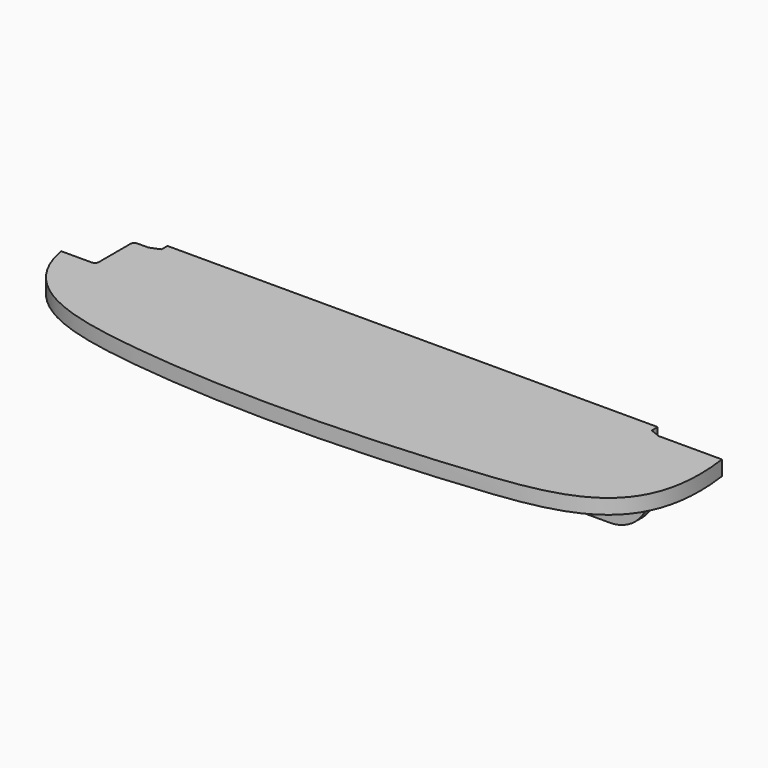
from build123d import *

# Parameters (mm, degrees)
F1_DEPTH = 19.05
F3_DEPTH = 25.4
F4_W     = 625.475
F4_H     = 11.1125
F5_DEPTH = 101.6
F6_R     = 50.8
F7_R     = 5.08


with BuildPart() as f1:
    # F0 (on Top) → F1 (new body)
    with BuildSketch(Plane.XY):
        with BuildLine():
            Line((398.4625, 0), (-398.4625, 0))
            Line((-398.4625, 0), (-398.4625, -75.40625))
            add(Edge.make_bspline(
                [(-398.4625, -75.40625), (-382.7767657486, -158.8698293815), (-186.1213914705, -212.4356276363), (207.7106026788, -201.6622700018), (427.1077817692, -162.9815576871), (398.4625, 0)],
                knots=[0.0603535709, 0.0603535709, 0.0603535709, 0.0603535709, 0.3014904815, 0.6985095185, 1, 1, 1, 1], degree=3))
        make_face()
    extrude(amount=F1_DEPTH)

    # F2 (on face) → F3 (cut)
    with BuildSketch(Plane.XY.offset(19.05)):
        Polygon((-322.1280574799, 0), (-398.4625, 0), (-398.4625, -75.40625), (-354.0125, -75.40625), (-354.0125, -14.684375), (-334.9625, -14.684375), (-322.2625, -9.525), align=None)
        Polygon((398.4625, 0), (382.8563850403, 0), (306.5219425201, 0), (306.6563850403, -9.525), (319.3563850403, -14.684375), (338.4063850403, -14.684375), (402.6769697666, -14.684375), align=None)
    extrude(amount=-F3_DEPTH, mode=Mode.SUBTRACT)

    # F7
    f7_edges = [f1.edges().sort_by_distance(p)[0] for p in [
        (-354.0125, -75.40625, 9.525),
        (-354.0125, -14.684375, 9.525),
    ]]
    fillet(f7_edges, radius=F7_R)


with BuildPart() as f5:
    # F4 (on Top) → F5 (new body)
    with BuildSketch(Plane.XY):
        with Locations((-7.8030574799, -5.55625)):
            Rectangle(F4_W, F4_H)
    extrude(amount=-F5_DEPTH)

    # F6
    f6_edges = [f5.edges().sort_by_distance(p)[0] for p in [
        (-320.540557, -5.55625, -101.6),
        (304.934443, -5.55625, -101.6),
    ]]
    fillet(f6_edges, radius=F6_R)


solid = Compound([f1.part, f5.part])
